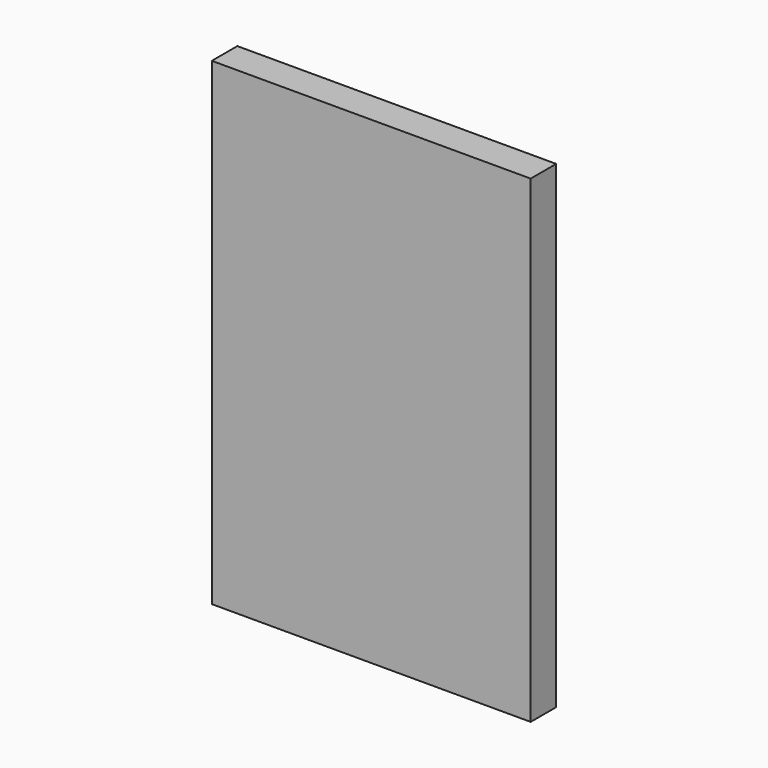
from build123d import *

# Parameters (mm, degrees)
F0_W     = 100
F0_H     = 150
F1_DEPTH = 10
F2_R     = 3.75
F3_DEPTH = 13


# Not quite as in the source:
# - a feature names something its author has since deleted; it is built from what else it names


with BuildPart() as f1:
    # F0 (on Front) → F1 (new body)
    with BuildSketch(Plane.XZ):
        with Locations((3.0784979463, 33.0328063236)):
            Rectangle(F0_W, F0_H)
    extrude(amount=F1_DEPTH)

    # F2 (on face) → F3 (join)
    with BuildSketch(Plane(origin=(0, 0, 0), x_dir=(-1, 0, 0), z_dir=(0, 1, 0))):
        with Locations((13.6121616811, 80.8424673975)):
            Circle(F2_R)
        with Locations((-4.3878383189, 80.8424673975)):
            Circle(F2_R)
        with Locations((-24.3878383189, 80.8424673975)):
            Circle(F2_R)
        with Locations((-24.3878383189, 58.8424673975)):
            Circle(F2_R)
        with Locations((-24.3878383189, 34.8424673975)):
            Circle(F2_R)
        with Locations((-24.3878383189, 8.8424673975)):
            Circle(F2_R)
        with Locations((-24.3878383189, -19.1575326025)):
            Circle(F2_R)
    extrude(amount=F3_DEPTH)


solid = f1.part
